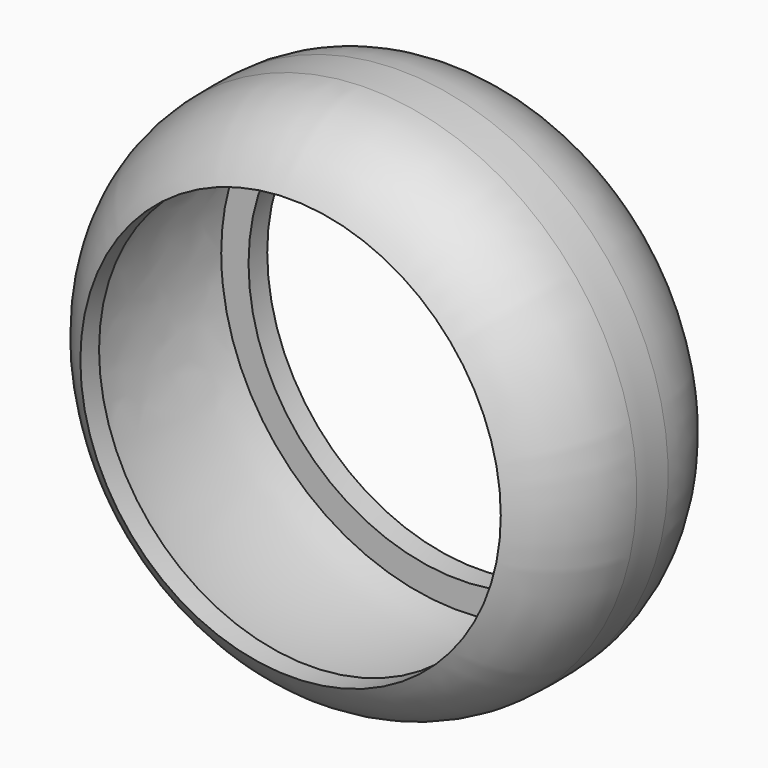
from build123d import *

# Parameters (mm, degrees)
F2_T = -1


# Not quite as in the source:
# - a fillet or chamfer that OpenCascade refuses, or shapes differently, is made with other operations: its cross-section is extruded or revolved along the edge and cut away or added


with BuildPart() as f1:
    # F0 (on Top) → F1 (revolve)
    with BuildSketch(Plane.XY):
        with BuildLine():
            Line((-9, -5), (-9, 5))
            Line((-9, 5), (-11, 5))
            ThreePointArc((-11, 5), (-11.5051025722, 0), (-11, -5))
            Line((-11, -5), (-9, -5))
        make_face()
    revolve(axis=Axis((0, -6.733, 0), (0, -1, 0)))

    # F2
    f2_openings = [f1.faces().sort_by_distance(p)[0] for p in [
        (9, 0, 0),
    ]]
    offset(amount=F2_T, openings=f2_openings, kind=Kind.INTERSECTION)

    # F3: fillet of radius 5 on 3 edges, made by hand

    # F3_s1 → F3_t2 (revolve, cut)
    with BuildSketch(Plane.XY):
        with BuildLine():
            ThreePointArc((-9, 5), (-10.7830276766, 3.2429528622), (-11.4909242519, 0.8418521191))
            Line((-11.4909242519, 0.8418521191), (-11.5908675386, 0.8452195276))
            ThreePointArc((-11.5908675386, 0.8452195276), (-11.4319769318, 2.9429465947), (-11.0979795897, 5.02))
            Line((-11.0979795897, 5.02), (-11, 5.1))
            ThreePointArc((-11, 5.1), (-10, 5.1), (-9.0501248017, 5.0865303661))
            Line((-9.0501248017, 5.0865303661), (-9, 5))
        make_face()
    revolve(axis=Axis((0, 5, 0), (0, -1, 0)), mode=Mode.SUBTRACT)

    # F3_s3 → F3_t4 (revolve, cut)
    with BuildSketch(Plane.XY):
        with BuildLine():
            ThreePointArc((-11.4909242519, -0.8418521191), (-10.7830276766, -3.2429528622), (-9, -5))
            Line((-9, -5), (-9.0501248017, -5.0865303661))
            ThreePointArc((-9.0501248017, -5.0865303661), (-10, -5.1), (-11, -5.1))
            Line((-11, -5.1), (-11.0979795897, -5.02))
            ThreePointArc((-11.0979795897, -5.02), (-11.4319769318, -2.9429465947), (-11.5908675386, -0.8452195276))
            Line((-11.5908675386, -0.8452195276), (-11.4909242519, -0.8418521191))
        make_face()
    revolve(axis=Axis((0, -5, 0), (0, -1, 0)), mode=Mode.SUBTRACT)


solid = f1.part
